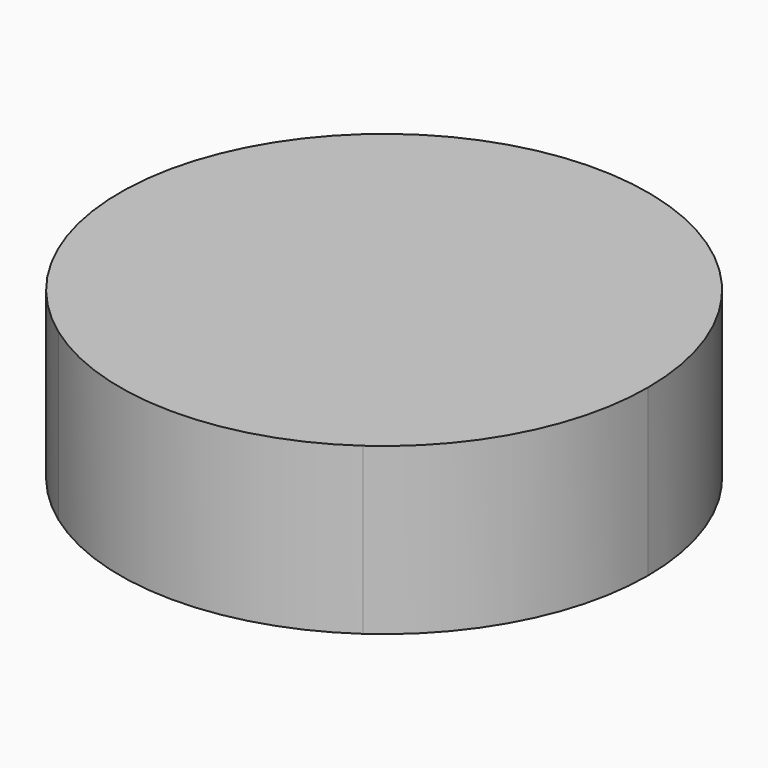
from build123d import *

# Parameters (mm, degrees)
F2_DEPTH = 19.36768


# Not quite as in the source:
# - a feature of the source that left no trace in its solid (it failed there, or was rolled back) is left out
# - the program builds the solid bodies; features that only make, move or delete a surface that nothing else refers to are left out


with BuildPart() as f2:
    # F0 (on Top) → F2 (new body)
    with BuildSketch(Plane.XY):
        with BuildLine():
            ThreePointArc((-4.863084816, 17.1141110558), (4.7921910677, 28.1431057658), (8.2721280354, 42.382246028))
            ThreePointArc((8.2721280354, 42.382246028), (-36.6726675985, 69.8596735008), (-40.6405812437, 17.3306402297))
            ThreePointArc((-40.6405812437, 17.3306402297), (-22.786398147, 11.5111205147), (-4.863084816, 17.1141110558))
        make_face()
    extrude(amount=F2_DEPTH)


solid = f2.part
